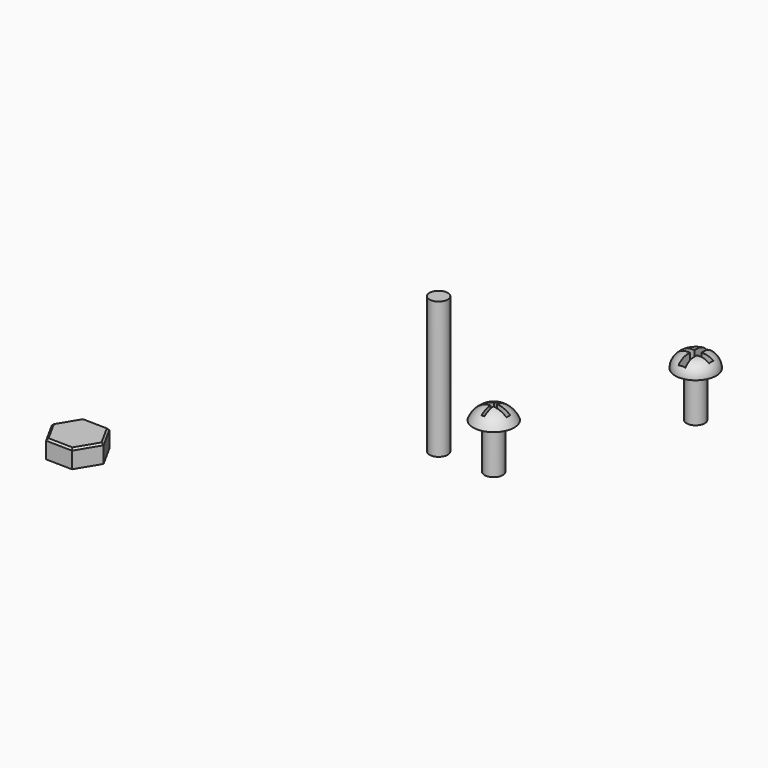
from build123d import *

# Parameters (mm, degrees)
F0_R      = 2
F1_DEPTH  = 30
F3_DEPTH  = 2
F6_R      = 2
F7_DEPTH  = 25
F8_R      = 2
F9_DEPTH  = 10
F10_R     = 4.5
F11_DEPTH = 3
F12_R     = 2.99999
F13_W     = 1.5
F13_H     = 3.1823935074
F13_H_2   = 1.2
F13_W_2   = 2.6515979143
F14_DEPTH = 2.41106
F15_SIZE  = 0.4
F19_START = -1
F19_DEPTH = 19.001


# Not quite as in the source:
# - a fillet or chamfer is up to 0.001 mm smaller than in the source, because OpenCascade refuses the exact size
# - the program builds the solid bodies; features that only make, move or delete a surface that nothing else refers to are left out


with BuildPart() as f1:
    # F0 (on Top) → F1 (new body)
    with BuildSketch(Plane.XY):
        Circle(F0_R)
    extrude(amount=F1_DEPTH)


with BuildPart() as f3:
    # F2 (on Top) → F3 (new body, symmetric)
    with BuildSketch(Plane.XY):
        Polygon((-44.3412244239, -36.4691410829), (-47.1302721521, -31.4139906298), (-52.9026847286, -31.3018015883), (-55.8860495767, -36.2447629999), (-53.0970018485, -41.2999134529), (-47.3245892721, -41.4121024944), align=None)
    extrude(amount=F3_DEPTH, both=True)

    # F6 (on face) → F7 (cut)
    with BuildSketch(Plane.XY):
        with Locations((-50.1136370003, -36.3569520414)):
            Circle(F6_R)
    extrude(amount=-F7_DEPTH, mode=Mode.SUBTRACT)

    # F15
    f15_edges = [f3.edges().sort_by_distance(p)[0] for p in [
        (-54.394367, -33.773282, 2),
        (-50.016478, -31.357896, 2),
        (-45.735748, -33.941566, 2),
        (-54.491526, -38.772338, 2),
        (-50.210796, -41.356008, 2),
        (-45.832907, -38.940622, 2),
    ]]
    chamfer(f15_edges, length=F15_SIZE)


with BuildPart() as f9:
    # F8 (on Top) → F9 (new body)
    with BuildSketch(Plane.XY):
        with Locations((27.0922463387, 36.6377010942)):
            Circle(F8_R)
    extrude(amount=F9_DEPTH)

    # F10 (on face) → F11 (join)
    with BuildSketch(Plane.XY.offset(10)):
        with Locations((27.0922463387, 36.6377010942)):
            Circle(F10_R)
    extrude(amount=F11_DEPTH)

    # F12 (radius 3 in the source; OpenCascade refuses exactly that, so slightly less here)
    f12_edges = [f9.edges().sort_by_distance(p)[0] for p in [
        (22.592246, 36.637701, 13),
    ]]
    fillet(f12_edges, radius=F12_R)

    # F13 (on face) → F14 (cut)
    with BuildSketch(Plane.XY.offset(13)):
        with Locations((27.0922463387, 34.4465043404)):
            Rectangle(F13_W, F13_H)
        with Locations((27.0922463387, 36.6377010942)):
            Rectangle(F13_W, F13_H_2)
        with Locations((29.1680452959, 36.6377010942)):
            Rectangle(F13_W_2, F13_H_2)
        with Locations((25.0164473816, 36.6377010942)):
            Rectangle(F13_W_2, F13_H_2)
        with Locations((27.0922463387, 38.8288978479)):
            Rectangle(F13_W, F13_H)
    extrude(amount=-F14_DEPTH, mode=Mode.SUBTRACT)


with BuildPart() as f17:
    # F16 (on Front) → F17 (revolve)
    with BuildSketch(Plane.XZ):
        with BuildLine():
            Line((10.083048013, 0), (12.083048013, 0))
            Line((12.083048013, 0), (12.083048013, 13))
            ThreePointArc((12.083048013, 13), (9.3788845564, 12.1812451849), (7.583048013, 10))
            Line((7.583048013, 10), (10.083048013, 10))
            Line((10.083048013, 10), (10.083048013, 0))
        make_face()
    revolve(axis=Axis((12.083048013, 0, 5.7094343938), (0, 0, -1)))

    # F18 (on face) → F19 (cut)
    with BuildSketch(Plane(origin=(0, 0, 10), x_dir=(1, 0, 0), z_dir=(0, 0, -1)).offset(F19_START)):
        with BuildLine():
            Line((12.4078653753, 1.9734471569), (12.4078653753, 2.9453942552))
            Line((12.4078653753, 2.9453942552), (11.7582306508, 2.9453942552))
            Line((11.7582306508, 2.9453942552), (11.7582306508, 1.9734471569))
            ThreePointArc((11.7582306508, 1.9734471569), (12.083048013, 2), (12.4078653753, 1.9734471569))
        make_face()
        with BuildLine():
            ThreePointArc((12.4078653753, -1.9734471569), (12.083048013, -2), (11.7582306508, -1.9734471569))
            Line((11.7582306508, -1.9734471569), (11.7582306508, -2.9453942552))
            Line((11.7582306508, -2.9453942552), (12.4078653753, -2.9453942552))
            Line((12.4078653753, -2.9453942552), (12.4078653753, -1.9734471569))
        make_face()
        with BuildLine():
            Line((15.3060089797, 0.5210122326), (14.0139924072, 0.5210122326))
            ThreePointArc((14.0139924072, 0.5210122326), (14.0657089508, 0.2627843333), (14.083048013, 0))
            ThreePointArc((14.083048013, 0), (14.0657089508, -0.2627843333), (14.0139924072, -0.5210122326))
            Line((14.0139924072, -0.5210122326), (15.3060089797, -0.5210122326))
            Line((15.3060089797, -0.5210122326), (15.3060089797, 0.5210122326))
        make_face()
        with BuildLine():
            ThreePointArc((10.1521036188, -0.5210122326), (10.083048013, 0), (10.1521036188, 0.5210122326))
            Line((10.1521036188, 0.5210122326), (8.8600870464, 0.5210122326))
            Line((8.8600870464, 0.5210122326), (8.8600870464, -0.5210122326))
            Line((8.8600870464, -0.5210122326), (10.1521036188, -0.5210122326))
        make_face()
        with BuildLine():
            Line((12.4078653753, 0.5210122326), (12.4078653753, 1.9734471569))
            ThreePointArc((12.4078653753, 1.9734471569), (12.083048013, 2), (11.7582306508, 1.9734471569))
            Line((11.7582306508, 1.9734471569), (11.7582306508, 0.5210122326))
            Line((11.7582306508, 0.5210122326), (10.1521036188, 0.5210122326))
            ThreePointArc((10.1521036188, 0.5210122326), (10.083048013, 0), (10.1521036188, -0.5210122326))
            Line((10.1521036188, -0.5210122326), (11.7582306508, -0.5210122326))
            Line((11.7582306508, -0.5210122326), (11.7582306508, -1.9734471569))
            ThreePointArc((11.7582306508, -1.9734471569), (12.083048013, -2), (12.4078653753, -1.9734471569))
            Line((12.4078653753, -1.9734471569), (12.4078653753, -0.5210122326))
            Line((12.4078653753, -0.5210122326), (14.0139924072, -0.5210122326))
            ThreePointArc((14.0139924072, -0.5210122326), (14.0657089508, -0.2627843333), (14.083048013, 0))
            ThreePointArc((14.083048013, 0), (14.0657089508, 0.2627843333), (14.0139924072, 0.5210122326))
            Line((14.0139924072, 0.5210122326), (12.4078653753, 0.5210122326))
        make_face()
    extrude(amount=-F19_DEPTH, mode=Mode.SUBTRACT)


solid = Compound([f1.part, f3.part, f9.part, f17.part])
